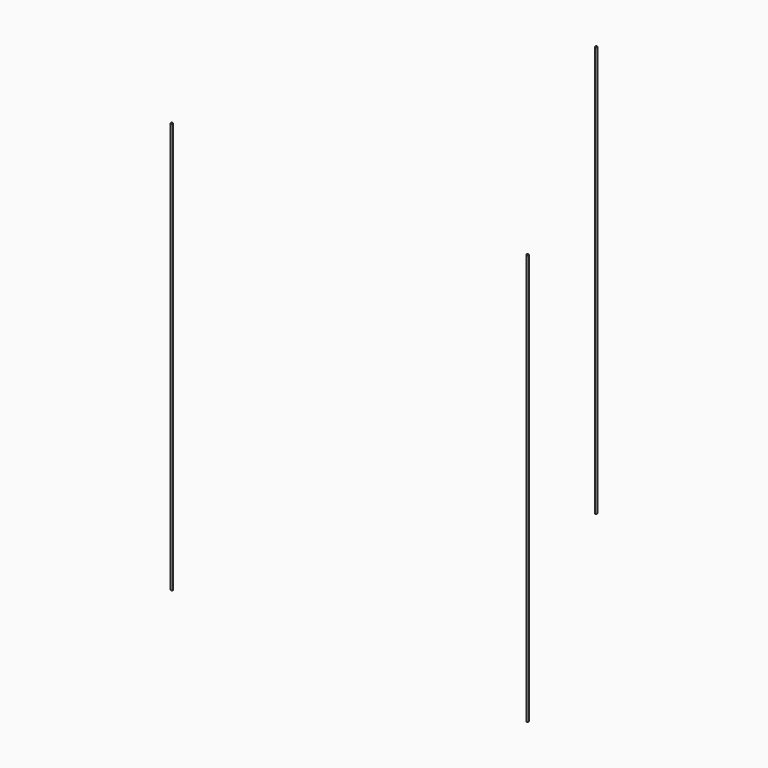
from build123d import *

# Parameters (mm, degrees)
F0_R            = 0.5
F1_DEPTH        = 200
F1_COPIES_COUNT = 3


# Not quite as in the source:
# - a pattern or mirror of a feature is missing from the dataset's text; its kind, count and spacing are read off the source's solid


with BuildPart() as f1:
    # F0 (on Top) → F1 (new body)
    with BuildSketch(Plane.XY):
        with Locations((0, 100)):
            Circle(F0_R)
    extrude(amount=F1_DEPTH)


with BuildPart() as f1_copies_1:
    # F1_copies: instance of F1
    add(f1.part.rotate(Axis((0, 0, 0), (0, 0, 1)), 1 * 360 / F1_COPIES_COUNT))


with BuildPart() as f1_copies_2:
    # F1_copies: instance of F1
    add(f1.part.rotate(Axis((0, 0, 0), (0, 0, 1)), 2 * 360 / F1_COPIES_COUNT))


solid = Compound([f1.part, f1_copies_1.part, f1_copies_2.part])
